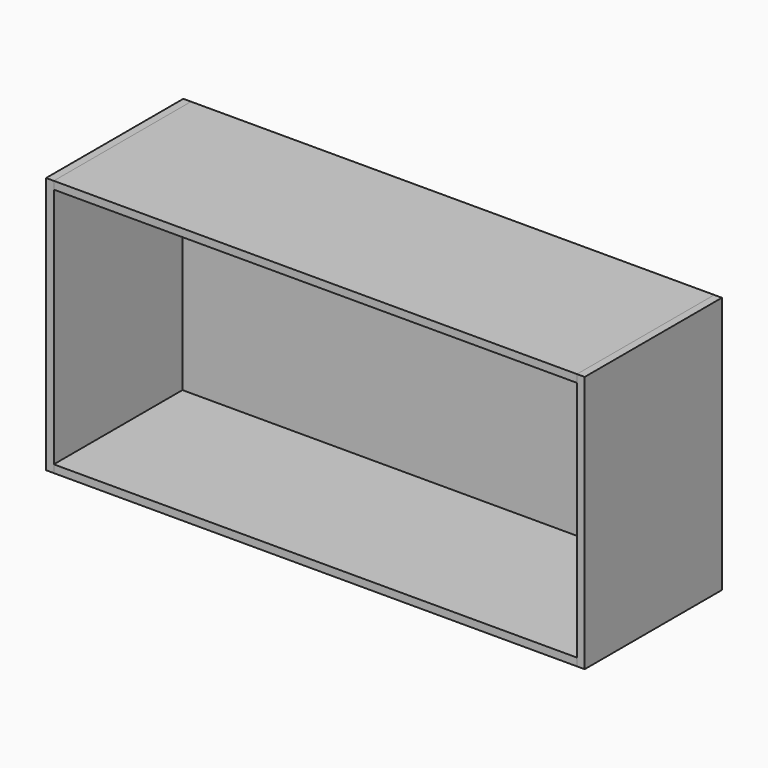
from build123d import *

# Parameters (mm, degrees)
F2_W          = 1220
F2_H          = 600
F3_DEPTH      = 5
F5_DEPTH      = 18
F8_DEPTH      = 12
F8_DEPTH_BACK = 3
F10_W         = 1220
F10_H         = 400
F11_DEPTH     = 18


# Not quite as in the source:
# - a feature names something its author has since deleted; it is built from what else it names


with BuildPart() as f3:
    # F2 (on Front) → F3 (new body)
    with BuildSketch(Plane.XZ):
        with Locations((628, 300)):
            Rectangle(F2_W, F2_H)
    extrude(amount=F3_DEPTH)


with BuildPart() as f5:
    # F4 (on Right) → F5 (new body)
    with BuildSketch(Plane.YZ):
        Polygon((0, 0), (20, 0), (20, 600), (-380, 600), (-380, 0), align=None)
    extrude(amount=F5_DEPTH)


with BuildPart() as f6_1:
    # F6: copy of F5
    add(f5.part.moved(Location((1238, 0, 0))))


with BuildPart() as f8:
    # F7 (on Top) → F8 (new body, two sides)
    with BuildSketch(Plane.XY) as f8_sk:
        Polygon((6.5949451849, 3), (3, 3), (3, 18), (-21, 18), (-21, -23), (3, -23), (3, -8), (6.5949451849, -8), align=None)
        Polygon((0, 15), (0, 0), (3.5949451849, 0), (3.5949451849, -5), (0, -5), (0, -20), (-18, -20), (-18, 15), align=None, mode=Mode.SUBTRACT)
        Polygon((3.5949451849, 0), (0, 0), (0, 15), (-18, 15), (-18, -20), (0, -20), (0, -5), (3.5949451849, -5), align=None)
    extrude(amount=F8_DEPTH)
    extrude(f8_sk.sketch, amount=-F8_DEPTH_BACK)

    # F9: cut F3, F5, F6_1
    add(f3.part, mode=Mode.SUBTRACT)
    add(f5.part, mode=Mode.SUBTRACT)
    add(f6_1.part, mode=Mode.SUBTRACT)


with BuildPart() as f11:
    # F10 (on Top) → F11 (new body)
    with BuildSketch(Plane.XY):
        with Locations((628, -180)):
            Rectangle(F10_W, F10_H)
    extrude(amount=F11_DEPTH)


with BuildPart() as f12_1:
    # F12: copy of F11
    add(f11.part.moved(Location((0, 0, 582))))


solid = Compound([f3.part, f5.part, f6_1.part, f8.part, f11.part, f12_1.part])
